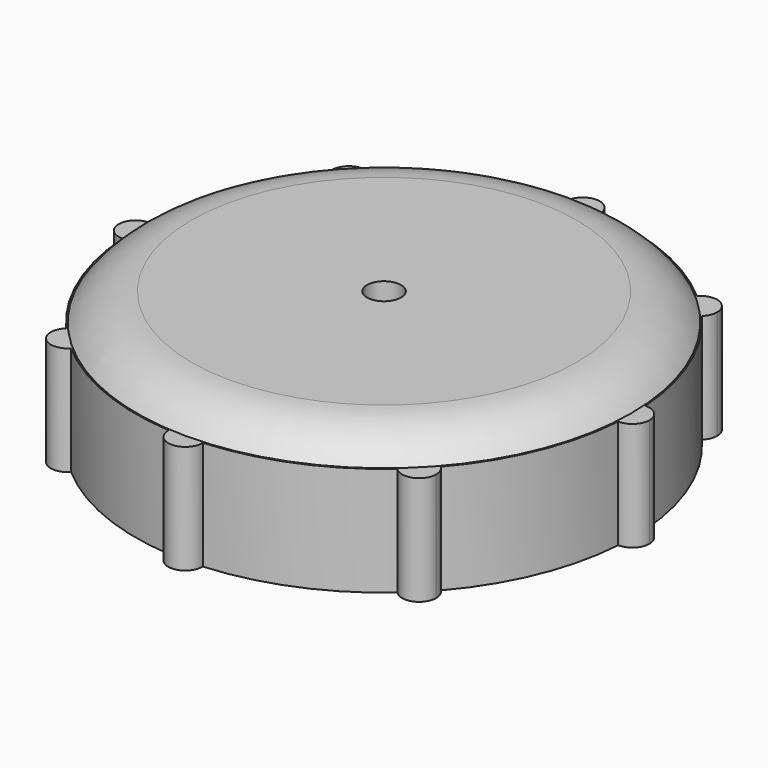
from build123d import *

# Parameters (mm, degrees)
F1_DEPTH = 8
F2_R     = 16.7410714552
F3_DEPTH = 4.8
F4_R     = 18.15
F5_DEPTH = 2
F7_R     = 1.25
F8_DEPTH = 25


# Not quite as in the source:
# - a fillet or chamfer that OpenCascade refuses, or shapes differently, is made with other operations: its cross-section is extruded or revolved along the edge and cut away or added


with BuildPart() as f1:
    # F0 (on Top) → F1 (new body)
    with BuildSketch(Plane.XY):
        with BuildLine():
            ThreePointArc((18.2071917808, -1.2492667675), (18.2392948054, -0.625), (18.25, 0))
            ThreePointArc((18.25, 0), (18.2392948054, 0.625), (18.2071917808, 1.2492667675))
            ThreePointArc((18.2071917808, 1.2492667675), (17, 0), (18.2071917808, -1.2492667675))
        make_face()
        with BuildLine():
            ThreePointArc((18.2071917808, 1.2492667675), (18.2392948054, 0.625), (18.25, 0))
            ThreePointArc((18.25, 0), (18.2392948054, -0.625), (18.2071917808, -1.2492667675))
            ThreePointArc((18.2071917808, -1.2492667675), (19.1186166375, -0.8988910596), (19.5, 0))
            ThreePointArc((19.5, 0), (19.1186166375, 0.8988910596), (18.2071917808, 1.2492667675))
        make_face()
        with BuildLine():
            ThreePointArc((18.2071917808, -1.2492667675), (17, 0), (18.2071917808, 1.2492667675))
            ThreePointArc((18.2071917808, 1.2492667675), (16.8608014683, 6.9839726407), (13.7577937774, 11.9910637718))
            ThreePointArc((13.7577937774, 11.9910637718), (12.0208152802, 12.0208152802), (11.9910637718, 13.7577937774))
            ThreePointArc((11.9910637718, 13.7577937774), (6.9839726407, 16.8608014683), (1.2492667675, 18.2071917808))
            ThreePointArc((1.2492667675, 18.2071917808), (0, 17), (-1.2492667675, 18.2071917808))
            ThreePointArc((-1.2492667675, 18.2071917808), (-6.9839726407, 16.8608014683), (-11.9910637718, 13.7577937774))
            ThreePointArc((-11.9910637718, 13.7577937774), (-11.7418265085, 13.3632051737), (-11.6546987567, 12.9046987567))
            ThreePointArc((-11.6546987567, 12.9046987567), (-12.406636901, 11.7582109076), (-13.7577937774, 11.9910637718))
            ThreePointArc((-13.7577937774, 11.9910637718), (-16.8608014683, 6.9839726407), (-18.2071917808, 1.2492667675))
            ThreePointArc((-18.2071917808, 1.2492667675), (-17.3511089404, 0.8686166375), (-17, 0))
            ThreePointArc((-17, 0), (-17.3511089404, -0.8686166375), (-18.2071917808, -1.2492667675))
            ThreePointArc((-18.2071917808, -1.2492667675), (-16.8608014683, -6.9839726407), (-13.7577937774, -11.9910637718))
            ThreePointArc((-13.7577937774, -11.9910637718), (-12.406636901, -11.7582109076), (-11.6546987567, -12.9046987567))
            ThreePointArc((-11.6546987567, -12.9046987567), (-11.7418265085, -13.3632051737), (-11.9910637718, -13.7577937774))
            ThreePointArc((-11.9910637718, -13.7577937774), (-6.9839726407, -16.8608014683), (-1.2492667675, -18.2071917808))
            ThreePointArc((-1.2492667675, -18.2071917808), (0, -17), (1.2492667675, -18.2071917808))
            ThreePointArc((1.2492667675, -18.2071917808), (6.9839726407, -16.8608014683), (11.9910637718, -13.7577937774))
            ThreePointArc((11.9910637718, -13.7577937774), (12.0208152802, -12.0208152802), (13.7577937774, -11.9910637718))
            ThreePointArc((13.7577937774, -11.9910637718), (16.8608014683, -6.9839726407), (18.2071917808, -1.2492667675))
        make_face()
        with BuildLine():
            ThreePointArc((11.9910637718, 13.7577937774), (12.0208152802, 12.0208152802), (13.7577937774, 11.9910637718))
            ThreePointArc((13.7577937774, 11.9910637718), (12.9046987567, 12.9046987567), (11.9910637718, 13.7577937774))
        make_face()
        with BuildLine():
            ThreePointArc((11.9910637718, 13.7577937774), (12.9046987567, 12.9046987567), (13.7577937774, 11.9910637718))
            ThreePointArc((13.7577937774, 11.9910637718), (14.0511866057, 12.406636901), (14.1546987567, 12.9046987567))
            ThreePointArc((14.1546987567, 12.9046987567), (13.3632051737, 14.0675710048), (11.9910637718, 13.7577937774))
        make_face()
        with BuildLine():
            ThreePointArc((14.1546987567, -12.9046987567), (14.0511866057, -12.406636901), (13.7577937774, -11.9910637718))
            ThreePointArc((13.7577937774, -11.9910637718), (12.9046987567, -12.9046987567), (11.9910637718, -13.7577937774))
            ThreePointArc((11.9910637718, -13.7577937774), (13.3632051737, -14.0675710048), (14.1546987567, -12.9046987567))
        make_face()
        with BuildLine():
            ThreePointArc((11.9910637718, -13.7577937774), (12.9046987567, -12.9046987567), (13.7577937774, -11.9910637718))
            ThreePointArc((13.7577937774, -11.9910637718), (12.0208152802, -12.0208152802), (11.9910637718, -13.7577937774))
        make_face()
        with BuildLine():
            ThreePointArc((-1.2492667675, 18.2071917808), (0, 17), (1.2492667675, 18.2071917808))
            ThreePointArc((1.2492667675, 18.2071917808), (0, 18.25), (-1.2492667675, 18.2071917808))
        make_face()
        with BuildLine():
            ThreePointArc((-1.2492667675, 18.2071917808), (0, 18.25), (1.2492667675, 18.2071917808))
            ThreePointArc((1.2492667675, 18.2071917808), (1.2498166784, 18.2285927509), (1.25, 18.25))
            ThreePointArc((1.25, 18.25), (-0.0214072491, 19.4998166784), (-1.2492667675, 18.2071917808))
        make_face()
        with BuildLine():
            ThreePointArc((1.25, -18.25), (1.2498166784, -18.2285927509), (1.2492667675, -18.2071917808))
            ThreePointArc((1.2492667675, -18.2071917808), (0, -18.25), (-1.2492667675, -18.2071917808))
            ThreePointArc((-1.2492667675, -18.2071917808), (-0.0214072491, -19.4998166784), (1.25, -18.25))
        make_face()
        with BuildLine():
            ThreePointArc((-1.2492667675, -18.2071917808), (0, -18.25), (1.2492667675, -18.2071917808))
            ThreePointArc((1.2492667675, -18.2071917808), (0, -17), (-1.2492667675, -18.2071917808))
        make_face()
        with BuildLine():
            ThreePointArc((-11.6546987567, 12.9046987567), (-11.7418265085, 13.3632051737), (-11.9910637718, 13.7577937774))
            ThreePointArc((-11.9910637718, 13.7577937774), (-12.9046987567, 12.9046987567), (-13.7577937774, 11.9910637718))
            ThreePointArc((-13.7577937774, 11.9910637718), (-12.406636901, 11.7582109076), (-11.6546987567, 12.9046987567))
        make_face()
        with BuildLine():
            ThreePointArc((-13.7577937774, 11.9910637718), (-12.9046987567, 12.9046987567), (-11.9910637718, 13.7577937774))
            ThreePointArc((-11.9910637718, 13.7577937774), (-13.7885822331, 13.7885822331), (-13.7577937774, 11.9910637718))
        make_face()
        with BuildLine():
            ThreePointArc((-13.7577937774, -11.9910637718), (-13.7885822331, -13.7885822331), (-11.9910637718, -13.7577937774))
            ThreePointArc((-11.9910637718, -13.7577937774), (-12.9046987567, -12.9046987567), (-13.7577937774, -11.9910637718))
        make_face()
        with BuildLine():
            ThreePointArc((-13.7577937774, -11.9910637718), (-12.9046987567, -12.9046987567), (-11.9910637718, -13.7577937774))
            ThreePointArc((-11.9910637718, -13.7577937774), (-11.7418265085, -13.3632051737), (-11.6546987567, -12.9046987567))
            ThreePointArc((-11.6546987567, -12.9046987567), (-12.406636901, -11.7582109076), (-13.7577937774, -11.9910637718))
        make_face()
        with BuildLine():
            ThreePointArc((-17, 0), (-17.3511089404, 0.8686166375), (-18.2071917808, 1.2492667675))
            ThreePointArc((-18.2071917808, 1.2492667675), (-18.25, 0), (-18.2071917808, -1.2492667675))
            ThreePointArc((-18.2071917808, -1.2492667675), (-17.3511089404, -0.8686166375), (-17, 0))
        make_face()
        with BuildLine():
            ThreePointArc((-18.2071917808, -1.2492667675), (-18.25, 0), (-18.2071917808, 1.2492667675))
            ThreePointArc((-18.2071917808, 1.2492667675), (-19.5, 0), (-18.2071917808, -1.2492667675))
        make_face()
    extrude(amount=F1_DEPTH)

    # F2 (on face) → F3 (cut)
    with BuildSketch(Plane(origin=(0, 0, 0), x_dir=(1, 0, 0), z_dir=(0, 0, -1))):
        Circle(F2_R)
    extrude(amount=-F3_DEPTH, mode=Mode.SUBTRACT)

    # F4 (on face) → F5 (join)
    with BuildSketch(Plane.XY.offset(8)):
        Circle(F4_R)
    extrude(amount=F5_DEPTH)

    # F6: fillet of radius 5 on 1 edges, made by hand

    # F6_s1 → F6_t2 (revolve, cut)
    with BuildSketch(Plane.XZ):
        with BuildLine():
            ThreePointArc((18.15, 8), (16.3860679775, 9.472135955), (14.15, 10))
            Line((14.15, 10), (18.15, 10))
            Line((18.15, 10), (18.15, 8))
        make_face()
    revolve(axis=Axis((0, 0, 10), (0, 0, 1)), mode=Mode.SUBTRACT)

    # F7 (on face) → F8 (cut)
    with BuildSketch(Plane(origin=(0, 0, 4.8), x_dir=(1, 0, 0), z_dir=(0, 0, -1))):
        Circle(F7_R)
    extrude(amount=-F8_DEPTH, mode=Mode.SUBTRACT)


solid = f1.part
